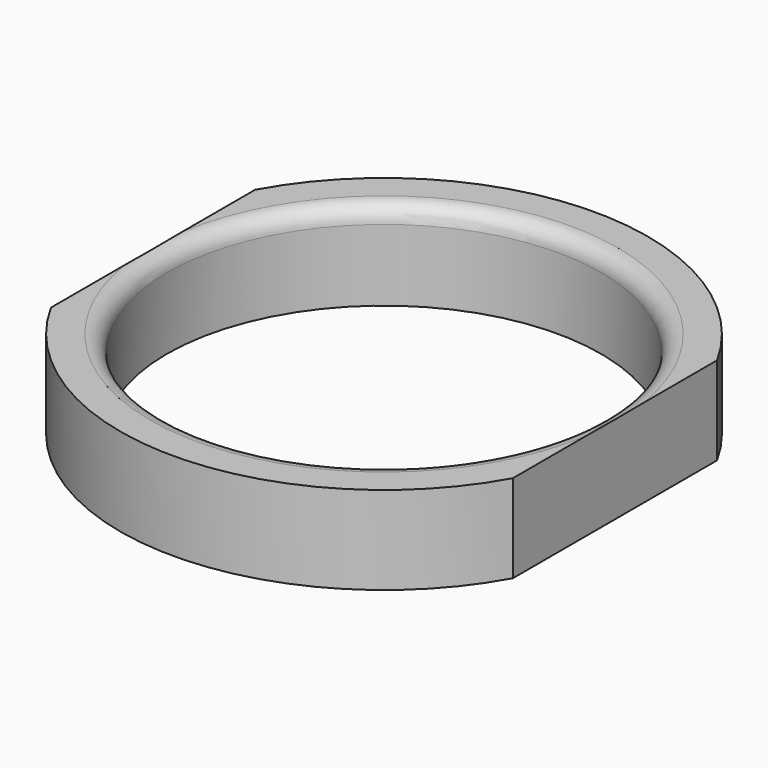
from build123d import *

# Parameters (mm, degrees)
F0_R     = 19.715
F1_DEPTH = 8


# Not quite as in the source:
# - a fillet or chamfer that OpenCascade refuses, or shapes differently, is made with other operations: its cross-section is extruded or revolved along the edge and cut away or added


with BuildPart() as f1:
    # F0 (on Top) → F1 (new body)
    with BuildSketch(Plane.XY):
        with BuildLine():
            Line((20.97, -11.5905435593), (20.97, 11.5905435593))
            ThreePointArc((20.97, 11.5905435593), (0, 23.96), (-20.97, 11.5905435593))
            Line((-20.97, 11.5905435593), (-20.97, -11.5905435593))
            ThreePointArc((-20.97, -11.5905435593), (0, -23.96), (20.97, -11.5905435593))
        make_face()
        Circle(F0_R, mode=Mode.SUBTRACT)
    extrude(amount=F1_DEPTH)

    # F2: fillet of radius 1.5 on 1 edges, made by hand

    # F2_s1 → F2_t2 (revolve, cut)
    with BuildSketch(Plane.XZ):
        with BuildLine():
            ThreePointArc((19.715, 6.5), (20.1543398282, 7.5606601718), (21.215, 8))
            Line((21.215, 8), (19.715, 8))
            Line((19.715, 8), (19.715, 6.5))
        make_face()
    revolve(axis=Axis((0, 0, 8), (0, 0, 1)), mode=Mode.SUBTRACT)


solid = f1.part
